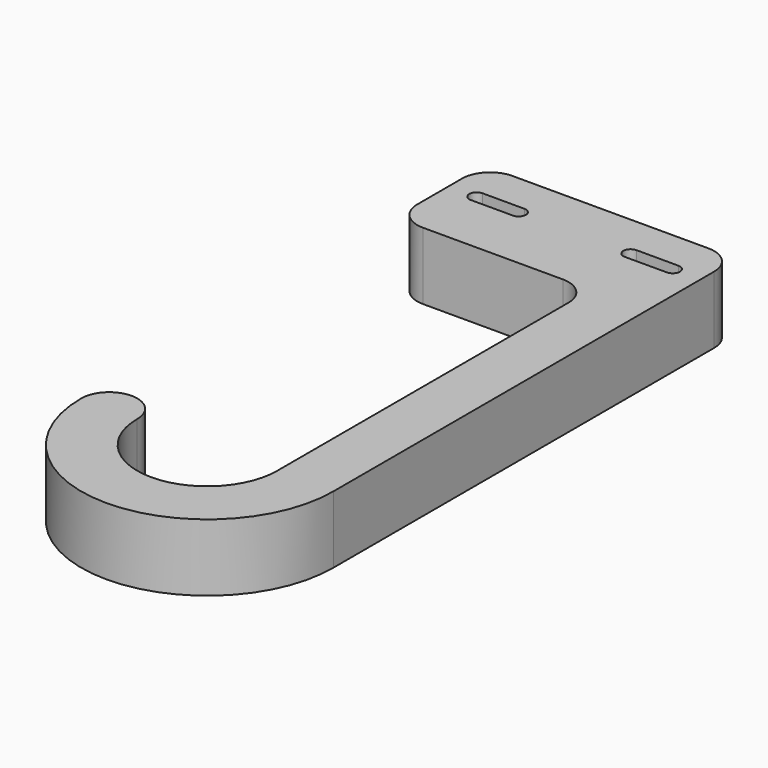
from build123d import *

# Parameters (mm, degrees)
F1_DEPTH = 3.81
F2_R     = 22.225
F3_DEPTH = 109
F4_DEPTH = 28.576


# Not quite as in the source:
# - an extrude ends at something that could not be found from the text; its depth is read off the source's solid
# - a pattern or mirror of a feature is missing from the dataset's text; its kind, count and spacing are read off the source's solid


with BuildPart() as f1:
    # F0 (on Top) → F1 (new body)
    with BuildSketch(Plane.XY):
        with BuildLine():
            ThreePointArc((7.9375, 0), (0, -7.9375), (-7.9375, 0))
            ThreePointArc((-7.9375, 0), (-8.8674359697, 2.2450640303), (-11.1125, 3.175))
            ThreePointArc((-11.1125, 3.175), (-13.3575640303, 2.2450640303), (-14.2875, 0))
            ThreePointArc((-14.2875, 0), (0, -14.2875), (14.2875, 0))
            Line((14.2875, 0), (14.2875, 53.975))
            ThreePointArc((14.2875, 53.975), (13.3575640303, 56.2200640303), (11.1125, 57.15))
            Line((11.1125, 57.15), (-11.1125, 57.15))
            ThreePointArc((-11.1125, 57.15), (-13.3575640303, 56.2200640303), (-14.2875, 53.975))
            Line((-14.2875, 53.975), (-14.2875, 47.625))
            ThreePointArc((-14.2875, 47.625), (-13.3575640303, 45.3799359697), (-11.1125, 44.45))
            Line((-11.1125, 44.45), (4.7625, 44.45))
            ThreePointArc((4.7625, 44.45), (7.0075640303, 43.5200640303), (7.9375, 41.275))
            Line((7.9375, 41.275), (7.9375, 0))
        make_face()
        with BuildLine():
            ThreePointArc((-11.1125, 51.2426083993), (-11.9398916007, 52.07), (-11.1125, 52.8973916007))
            Line((-11.1125, 52.8973916007), (-6.3490160938, 52.8936081389))
            ThreePointArc((-6.3490160938, 52.8936081389), (-5.5241718233, 52.0677805671), (-6.3496717582, 51.2426083993))
            Line((-6.3496717582, 51.2426083993), (-11.1125, 51.2426083993))
        make_face(mode=Mode.SUBTRACT)
        with BuildLine():
            ThreePointArc((11.1133453348, 52.8905930346), (11.93309347, 52.07), (11.1133453348, 51.2494069654))
            Line((11.1133453348, 51.2494069654), (6.35, 51.2445))
            ThreePointArc((6.35, 51.2445), (5.5245, 52.07), (6.35, 52.8955))
            Line((6.35, 52.8955), (11.1133453348, 52.8905930346))
        make_face(mode=Mode.SUBTRACT)
    extrude(amount=F1_DEPTH)

    # F1_copies: F1 across plane


with BuildPart() as f1_1:
    add(f1.part)
    add(f1.part.mirror(Plane.XY.offset(3.81)))

    # F2 (on face) → F3 (cut, through all)
    with BuildSketch(Plane(origin=(-14.2875, 0, 0), x_dir=(0, -1, 0), z_dir=(-1, 0, 0))):
        with Locations((79.121, 3.81)):
            Circle(F2_R)
        with BuildLine():
            ThreePointArc((-57.15, 0.4595098866), (-56.9595909744, 2.1299479175), (-56.896, 3.81))
            ThreePointArc((-56.896, 3.81), (-101.2824090256, 5.4900520825), (-57.15, 0.4595098866))
        make_face()
    extrude(amount=F3_DEPTH, mode=Mode.SUBTRACT)

    # F2 (on face) → F4 (cut, through all)
    with BuildSketch(Plane(origin=(-14.2875, 0, 0), x_dir=(0, -1, 0), z_dir=(-1, 0, 0))):
        with Locations((79.121, 3.81)):
            Circle(F2_R)
        with BuildLine():
            ThreePointArc((-57.15, 0.4595098866), (-56.9595909744, 2.1299479175), (-56.896, 3.81))
            ThreePointArc((-56.896, 3.81), (-101.2824090256, 5.4900520825), (-57.15, 0.4595098866))
        make_face()
    extrude(amount=-F4_DEPTH, mode=Mode.SUBTRACT)


solid = f1_1.part
